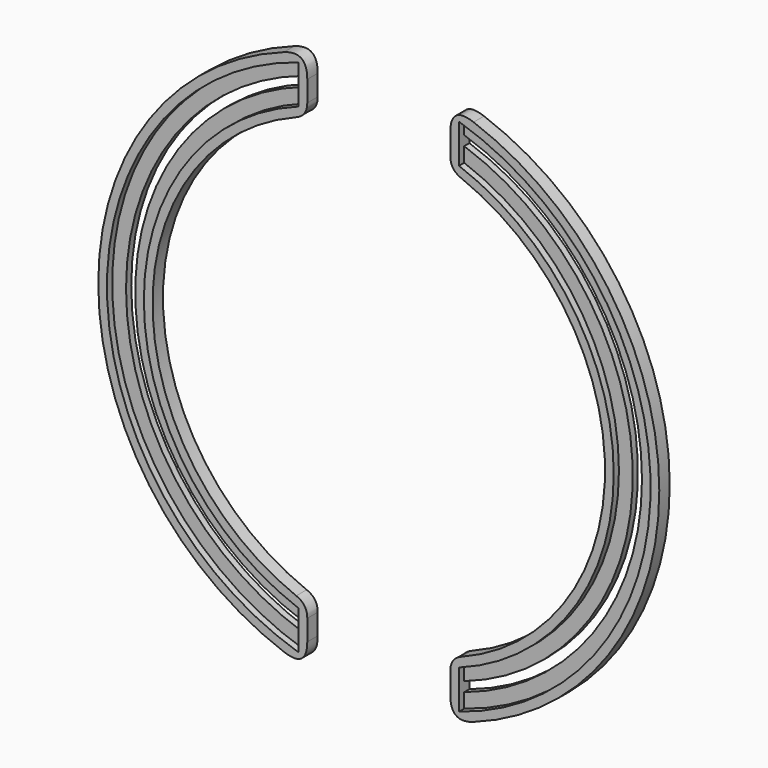
from build123d import *

# Parameters (mm, degrees)
F1_DEPTH      = 1.5
F2_DEPTH      = 3
F3_T1_DEPTH   = 31.0210256648
F3_T3_DEPTH   = 17.0194710076
F3_2_T1_DEPTH = 31.0210256648
F3_2_T3_DEPTH = 17.0194710075


# Not quite as in the source:
# - a fillet or chamfer that OpenCascade refuses, or shapes differently, is made with other operations: its cross-section is extruded or revolved along the edge and cut away or added


with BuildPart() as f1:
    # F0 (on Front) → F1 (new body)
    with BuildSketch(Plane.XZ):
        with BuildLine():
            ThreePointArc((-18.4309218526, 56.3415860789), (-17.4336374643, 56.6581105137), (-16.4309218526, 56.95698385))
            Line((-16.4309218526, 56.95698385), (-16.4309218526, 60.2544953802))
            ThreePointArc((-16.4309218526, 60.2544953802), (-17.433345569, 59.972142439), (-18.4309218526, 59.6731139301))
            Line((-18.4309218526, 59.6731139301), (-18.4309218526, 56.3415860789))
        make_face()
        with BuildLine():
            ThreePointArc((-18.4309218526, -56.3415860789), (-59.2796187759, 0), (-18.4309218526, 56.3415860789))
            Line((-18.4309218526, 56.3415860789), (-18.4309218526, 59.6731139301))
            ThreePointArc((-18.4309218526, 59.6731139301), (-62.4546187759, 0), (-18.4309218526, -59.6731139301))
            Line((-18.4309218526, -59.6731139301), (-18.4309218526, -56.3415860789))
        make_face()
        with BuildLine():
            ThreePointArc((-16.4309218526, -56.95698385), (-17.4336374643, -56.6581105137), (-18.4309218526, -56.3415860789))
            Line((-18.4309218526, -56.3415860789), (-18.4309218526, -59.6731139301))
            ThreePointArc((-18.4309218526, -59.6731139301), (-17.433345569, -59.972142439), (-16.4309218526, -60.2544953802))
            Line((-16.4309218526, -60.2544953802), (-16.4309218526, -56.95698385))
        make_face()
    extrude(amount=F1_DEPTH)



with BuildPart() as f1b:
    # F0 (on Front) → F1, piece 2 (new body)
    with BuildSketch(Plane.XZ):
        with BuildLine():
            ThreePointArc((-18.4309218526, 50.7441040985), (-17.4342611615, 51.0951026895), (-16.4309218526, 51.4265280587))
            Line((-16.4309218526, 51.4265280587), (-16.4309218526, 54.7502492451))
            ThreePointArc((-16.4309218526, 54.7502492451), (-17.4338634076, 54.4391898544), (-18.4309218526, 54.1097597942))
            Line((-18.4309218526, 54.1097597942), (-18.4309218526, 50.7441040985))
        make_face()
        with BuildLine():
            ThreePointArc((-18.4309218526, -50.7441040985), (-53.9876187759, 0), (-18.4309218526, 50.7441040985))
            Line((-18.4309218526, 50.7441040985), (-18.4309218526, 54.1097597942))
            ThreePointArc((-18.4309218526, 54.1097597942), (-57.1626187759, 0), (-18.4309218526, -54.1097597942))
            Line((-18.4309218526, -54.1097597942), (-18.4309218526, -50.7441040985))
        make_face()
        with BuildLine():
            ThreePointArc((-16.4309218526, -51.4265280587), (-17.4342611615, -51.0951026895), (-18.4309218526, -50.7441040985))
            Line((-18.4309218526, -50.7441040985), (-18.4309218526, -54.1097597942))
            ThreePointArc((-18.4309218526, -54.1097597942), (-17.4338634076, -54.4391898544), (-16.4309218526, -54.7502492451))
            Line((-16.4309218526, -54.7502492451), (-16.4309218526, -51.4265280587))
        make_face()
    extrude(amount=F1_DEPTH)


with BuildPart() as f1c:
    # F0 (on Front) → F1, piece 3 (new body)
    with BuildSketch(Plane.XZ):
        with BuildLine():
            ThreePointArc((18.4309218526, -56.3415860789), (17.4336374643, -56.6581105137), (16.4309218526, -56.95698385))
            Line((16.4309218526, -56.95698385), (16.4309218526, -60.2544953802))
            ThreePointArc((16.4309218526, -60.2544953802), (17.433345569, -59.972142439), (18.4309218526, -59.6731139301))
            Line((18.4309218526, -59.6731139301), (18.4309218526, -56.3415860789))
        make_face()
        with BuildLine():
            ThreePointArc((18.4309218526, 56.3415860789), (59.2796187759, 0), (18.4309218526, -56.3415860789))
            Line((18.4309218526, -56.3415860789), (18.4309218526, -59.6731139301))
            ThreePointArc((18.4309218526, -59.6731139301), (62.4546187759, 0), (18.4309218526, 59.6731139301))
            Line((18.4309218526, 59.6731139301), (18.4309218526, 56.3415860789))
        make_face()
        with BuildLine():
            ThreePointArc((16.4309218526, 56.95698385), (17.4336374643, 56.6581105137), (18.4309218526, 56.3415860789))
            Line((18.4309218526, 56.3415860789), (18.4309218526, 59.6731139301))
            ThreePointArc((18.4309218526, 59.6731139301), (17.433345569, 59.972142439), (16.4309218526, 60.2544953802))
            Line((16.4309218526, 60.2544953802), (16.4309218526, 56.95698385))
        make_face()
    extrude(amount=F1_DEPTH)



with BuildPart() as f1d:
    # F0 (on Front) → F1, piece 4 (new body)
    with BuildSketch(Plane.XZ):
        with BuildLine():
            ThreePointArc((18.4309218526, -50.7441040985), (17.4342611615, -51.0951026895), (16.4309218526, -51.4265280587))
            Line((16.4309218526, -51.4265280587), (16.4309218526, -54.7502492451))
            ThreePointArc((16.4309218526, -54.7502492451), (17.4338634076, -54.4391898544), (18.4309218526, -54.1097597942))
            Line((18.4309218526, -54.1097597942), (18.4309218526, -50.7441040985))
        make_face()
        with BuildLine():
            ThreePointArc((18.4309218526, 50.7441040985), (53.9876187759, 0), (18.4309218526, -50.7441040985))
            Line((18.4309218526, -50.7441040985), (18.4309218526, -54.1097597942))
            ThreePointArc((18.4309218526, -54.1097597942), (57.1626187759, 0), (18.4309218526, 54.1097597942))
            Line((18.4309218526, 54.1097597942), (18.4309218526, 50.7441040985))
        make_face()
        with BuildLine():
            ThreePointArc((16.4309218526, 51.4265280587), (17.4342611615, 51.0951026895), (18.4309218526, 50.7441040985))
            Line((18.4309218526, 50.7441040985), (18.4309218526, 54.1097597942))
            ThreePointArc((18.4309218526, 54.1097597942), (17.4338634076, 54.4391898544), (16.4309218526, 54.7502492451))
            Line((16.4309218526, 54.7502492451), (16.4309218526, 51.4265280587))
        make_face()
    extrude(amount=F1_DEPTH)


with BuildPart() as f1_1:
    add(f1.part)

    add(f1b.part)  # F2 merges F1b
    # F0 (on Front) → F2 (join)
    with BuildSketch(Plane.XZ):
        with BuildLine():
            ThreePointArc((-18.4309218526, 59.6731139301), (-17.433345569, 59.972142439), (-16.4309218526, 60.2544953802))
            Line((-16.4309218526, 60.2544953802), (-16.4309218526, 62.3251368921))
            ThreePointArc((-16.4309218526, 62.3251368921), (-17.4331857663, 62.0522514949), (-18.4309218526, 61.7632496005))
            Line((-18.4309218526, 61.7632496005), (-18.4309218526, 59.6731139301))
        make_face()
        with BuildLine():
            ThreePointArc((-18.4309218526, -59.6731139301), (-62.4546187759, 0), (-18.4309218526, 59.6731139301))
            Line((-18.4309218526, 59.6731139301), (-18.4309218526, 61.7632496005))
            ThreePointArc((-18.4309218526, 61.7632496005), (-64.4546187759, 0), (-18.4309218526, -61.7632496005))
            Line((-18.4309218526, -61.7632496005), (-18.4309218526, -59.6731139301))
        make_face()
        with BuildLine():
            ThreePointArc((-16.4309218526, -60.2544953802), (-17.433345569, -59.972142439), (-18.4309218526, -59.6731139301))
            Line((-18.4309218526, -59.6731139301), (-18.4309218526, -61.7632496005))
            ThreePointArc((-18.4309218526, -61.7632496005), (-17.4331857663, -62.0522514949), (-16.4309218526, -62.3251368921))
            Line((-16.4309218526, -62.3251368921), (-16.4309218526, -60.2544953802))
        make_face()
        with BuildLine():
            Line((-16.4309218526, 49.3227869556), (-16.4309218526, 51.4265280587))
            ThreePointArc((-16.4309218526, 51.4265280587), (-17.4342611615, 51.0951026895), (-18.4309218526, 50.7441040985))
            Line((-18.4309218526, 50.7441040985), (-18.4309218526, 48.6108385615))
            ThreePointArc((-18.4309218526, 48.6108385615), (-17.4345563253, 48.9770226916), (-16.4309218526, 49.3227869556))
        make_face()
        with BuildLine():
            Line((-18.4309218526, 48.6108385615), (-18.4309218526, 50.7441040985))
            ThreePointArc((-18.4309218526, 50.7441040985), (-53.9876187759, 0), (-18.4309218526, -50.7441040985))
            Line((-18.4309218526, -50.7441040985), (-18.4309218526, -48.6108385615))
            ThreePointArc((-18.4309218526, -48.6108385615), (-51.9876187759, 0), (-18.4309218526, 48.6108385615))
        make_face()
        with BuildLine():
            Line((-18.4309218526, -48.6108385615), (-18.4309218526, -50.7441040985))
            ThreePointArc((-18.4309218526, -50.7441040985), (-17.4342611615, -51.0951026895), (-16.4309218526, -51.4265280587))
            Line((-16.4309218526, -51.4265280587), (-16.4309218526, -49.3227869556))
            ThreePointArc((-16.4309218526, -49.3227869556), (-17.4345563253, -48.9770226916), (-18.4309218526, -48.6108385615))
        make_face()
        with BuildLine():
            ThreePointArc((-18.4309218526, 54.1097597942), (-17.4338634076, 54.4391898544), (-16.4309218526, 54.7502492451))
            Line((-16.4309218526, 54.7502492451), (-16.4309218526, 56.95698385))
            ThreePointArc((-16.4309218526, 56.95698385), (-17.4336374643, 56.6581105137), (-18.4309218526, 56.3415860789))
            Line((-18.4309218526, 56.3415860789), (-18.4309218526, 54.1097597942))
        make_face()
        with BuildLine():
            ThreePointArc((-18.4309218526, 50.7441040985), (-17.4342611615, 51.0951026895), (-16.4309218526, 51.4265280587))
            Line((-16.4309218526, 51.4265280587), (-16.4309218526, 54.7502492451))
            ThreePointArc((-16.4309218526, 54.7502492451), (-17.4338634076, 54.4391898544), (-18.4309218526, 54.1097597942))
            Line((-18.4309218526, 54.1097597942), (-18.4309218526, 50.7441040985))
        make_face()
        with BuildLine():
            ThreePointArc((-18.4309218526, 56.3415860789), (-17.4336374643, 56.6581105137), (-16.4309218526, 56.95698385))
            Line((-16.4309218526, 56.95698385), (-16.4309218526, 60.2544953802))
            ThreePointArc((-16.4309218526, 60.2544953802), (-17.433345569, 59.972142439), (-18.4309218526, 59.6731139301))
            Line((-18.4309218526, 59.6731139301), (-18.4309218526, 56.3415860789))
        make_face()
        with BuildLine():
            ThreePointArc((-16.4309218526, -51.4265280587), (-17.4342611615, -51.0951026895), (-18.4309218526, -50.7441040985))
            Line((-18.4309218526, -50.7441040985), (-18.4309218526, -54.1097597942))
            ThreePointArc((-18.4309218526, -54.1097597942), (-17.4338634076, -54.4391898544), (-16.4309218526, -54.7502492451))
            Line((-16.4309218526, -54.7502492451), (-16.4309218526, -51.4265280587))
        make_face()
        with BuildLine():
            ThreePointArc((-16.4309218526, -54.7502492451), (-17.4338634076, -54.4391898544), (-18.4309218526, -54.1097597942))
            Line((-18.4309218526, -54.1097597942), (-18.4309218526, -56.3415860789))
            ThreePointArc((-18.4309218526, -56.3415860789), (-17.4336374643, -56.6581105137), (-16.4309218526, -56.95698385))
            Line((-16.4309218526, -56.95698385), (-16.4309218526, -54.7502492451))
        make_face()
        with BuildLine():
            ThreePointArc((-16.4309218526, -56.95698385), (-17.4336374643, -56.6581105137), (-18.4309218526, -56.3415860789))
            Line((-18.4309218526, -56.3415860789), (-18.4309218526, -59.6731139301))
            ThreePointArc((-18.4309218526, -59.6731139301), (-17.433345569, -59.972142439), (-16.4309218526, -60.2544953802))
            Line((-16.4309218526, -60.2544953802), (-16.4309218526, -56.95698385))
        make_face()
    extrude(amount=F2_DEPTH)

    # F3#2: fillet of radius 4 on 4 edges, made by hand

    # F3_2_s2 → F3_2_t1 (cut)
    with BuildSketch(Plane.XZ.offset(-14.0105128324)):
        with BuildLine():
            add(Edge.make_bspline(
                [(-21.7827406063, -60.6622625133), (-16.4309218526, -62.5840055353), (-16.4309218526, -56.8976129869)],
                knots=[0, 0, 0, 1, 1, 1], degree=2, weights=[1, 1, 1]))
            Line((-16.4309218526, -56.8976129869), (-16.4309218526, -62.3251368921))
            ThreePointArc((-16.4309218526, -62.3251368921), (-19.1249127431, -61.5518935056), (-21.7827406063, -60.6622625133))
        make_face()
        with BuildLine():
            add(Edge.make_bspline(
                [(-16.4309218526, 56.8976129868), (-16.4309218526, 62.5840055353), (-21.7827406063, 60.6622625133)],
                knots=[0, 0, 0, 1, 1, 1], degree=2, weights=[1, 1, 1]))
            ThreePointArc((-21.7827406063, 60.6622625133), (-19.1249127431, 61.5518935056), (-16.4309218526, 62.3251368921))
            Line((-16.4309218526, 62.3251368921), (-16.4309218526, 56.8976129868))
        make_face()
    extrude(amount=F3_2_T1_DEPTH, mode=Mode.SUBTRACT)

    # F3_2_s4 → F3_2_t3 (cut)
    with BuildSketch(Plane.XZ.offset(-7.0097355038)):
        with BuildLine():
            add(Edge.make_bspline(
                [(-16.4309218526, -52.1266811571), (-16.4309218526, -49.3981976907), (-18.9712475675, -48.4025234024)],
                knots=[0, 0, 0, 1, 1, 1], degree=2, weights=[1, 1, 1]))
            ThreePointArc((-18.9712475675, -48.4025234024), (-17.7070641599, -48.8791610487), (-16.4309218526, -49.3227869556))
            Line((-16.4309218526, -49.3227869556), (-16.4309218526, -52.1266811571))
        make_face()
        with BuildLine():
            add(Edge.make_bspline(
                [(-16.4309218526, 52.1266811571), (-16.4309218526, 49.3981976907), (-18.9712475675, 48.4025234025)],
                knots=[0, 0, 0, 1, 1, 1], degree=2, weights=[1, 1, 1]))
            ThreePointArc((-18.9712475675, 48.4025234025), (-17.7070641599, 48.8791610487), (-16.4309218526, 49.3227869556))
            Line((-16.4309218526, 49.3227869556), (-16.4309218526, 52.1266811571))
        make_face()
    extrude(amount=F3_2_T3_DEPTH, mode=Mode.SUBTRACT)


with BuildPart() as f1c_1:
    add(f1c.part)

    add(f1d.part)  # F2#2 merges F1d
    # F0 (on Front) → F2, piece 2 (join)
    with BuildSketch(Plane.XZ):
        with BuildLine():
            Line((16.4309218526, -49.3227869556), (16.4309218526, -51.4265280587))
            ThreePointArc((16.4309218526, -51.4265280587), (17.4342611615, -51.0951026895), (18.4309218526, -50.7441040985))
            Line((18.4309218526, -50.7441040985), (18.4309218526, -48.6108385615))
            ThreePointArc((18.4309218526, -48.6108385615), (17.4345563253, -48.9770226916), (16.4309218526, -49.3227869556))
        make_face()
        with BuildLine():
            Line((18.4309218526, -48.6108385615), (18.4309218526, -50.7441040985))
            ThreePointArc((18.4309218526, -50.7441040985), (53.9876187759, 0), (18.4309218526, 50.7441040985))
            Line((18.4309218526, 50.7441040985), (18.4309218526, 48.6108385615))
            ThreePointArc((18.4309218526, 48.6108385615), (51.9876187759, 0), (18.4309218526, -48.6108385615))
        make_face()
        with BuildLine():
            Line((18.4309218526, 48.6108385615), (18.4309218526, 50.7441040985))
            ThreePointArc((18.4309218526, 50.7441040985), (17.4342611615, 51.0951026895), (16.4309218526, 51.4265280587))
            Line((16.4309218526, 51.4265280587), (16.4309218526, 49.3227869556))
            ThreePointArc((16.4309218526, 49.3227869556), (17.4345563253, 48.9770226916), (18.4309218526, 48.6108385615))
        make_face()
        with BuildLine():
            ThreePointArc((18.4309218526, -59.6731139301), (17.433345569, -59.972142439), (16.4309218526, -60.2544953802))
            Line((16.4309218526, -60.2544953802), (16.4309218526, -62.3251368921))
            ThreePointArc((16.4309218526, -62.3251368921), (17.4331857663, -62.0522514949), (18.4309218526, -61.7632496005))
            Line((18.4309218526, -61.7632496005), (18.4309218526, -59.6731139301))
        make_face()
        with BuildLine():
            ThreePointArc((18.4309218526, 59.6731139301), (62.4546187759, 0), (18.4309218526, -59.6731139301))
            Line((18.4309218526, -59.6731139301), (18.4309218526, -61.7632496005))
            ThreePointArc((18.4309218526, -61.7632496005), (64.4546187759, 0), (18.4309218526, 61.7632496005))
            Line((18.4309218526, 61.7632496005), (18.4309218526, 59.6731139301))
        make_face()
        with BuildLine():
            ThreePointArc((16.4309218526, 60.2544953802), (17.433345569, 59.972142439), (18.4309218526, 59.6731139301))
            Line((18.4309218526, 59.6731139301), (18.4309218526, 61.7632496005))
            ThreePointArc((18.4309218526, 61.7632496005), (17.4331857663, 62.0522514949), (16.4309218526, 62.3251368921))
            Line((16.4309218526, 62.3251368921), (16.4309218526, 60.2544953802))
        make_face()
        with BuildLine():
            ThreePointArc((16.4309218526, 54.7502492451), (17.4338634076, 54.4391898544), (18.4309218526, 54.1097597942))
            Line((18.4309218526, 54.1097597942), (18.4309218526, 56.3415860789))
            ThreePointArc((18.4309218526, 56.3415860789), (17.4336374643, 56.6581105137), (16.4309218526, 56.95698385))
            Line((16.4309218526, 56.95698385), (16.4309218526, 54.7502492451))
        make_face()
        with BuildLine():
            ThreePointArc((16.4309218526, 56.95698385), (17.4336374643, 56.6581105137), (18.4309218526, 56.3415860789))
            Line((18.4309218526, 56.3415860789), (18.4309218526, 59.6731139301))
            ThreePointArc((18.4309218526, 59.6731139301), (17.433345569, 59.972142439), (16.4309218526, 60.2544953802))
            Line((16.4309218526, 60.2544953802), (16.4309218526, 56.95698385))
        make_face()
        with BuildLine():
            ThreePointArc((16.4309218526, 51.4265280587), (17.4342611615, 51.0951026895), (18.4309218526, 50.7441040985))
            Line((18.4309218526, 50.7441040985), (18.4309218526, 54.1097597942))
            ThreePointArc((18.4309218526, 54.1097597942), (17.4338634076, 54.4391898544), (16.4309218526, 54.7502492451))
            Line((16.4309218526, 54.7502492451), (16.4309218526, 51.4265280587))
        make_face()
        with BuildLine():
            ThreePointArc((18.4309218526, -54.1097597942), (17.4338634076, -54.4391898544), (16.4309218526, -54.7502492451))
            Line((16.4309218526, -54.7502492451), (16.4309218526, -56.95698385))
            ThreePointArc((16.4309218526, -56.95698385), (17.4336374643, -56.6581105137), (18.4309218526, -56.3415860789))
            Line((18.4309218526, -56.3415860789), (18.4309218526, -54.1097597942))
        make_face()
        with BuildLine():
            ThreePointArc((18.4309218526, -50.7441040985), (17.4342611615, -51.0951026895), (16.4309218526, -51.4265280587))
            Line((16.4309218526, -51.4265280587), (16.4309218526, -54.7502492451))
            ThreePointArc((16.4309218526, -54.7502492451), (17.4338634076, -54.4391898544), (18.4309218526, -54.1097597942))
            Line((18.4309218526, -54.1097597942), (18.4309218526, -50.7441040985))
        make_face()
        with BuildLine():
            ThreePointArc((18.4309218526, -56.3415860789), (17.4336374643, -56.6581105137), (16.4309218526, -56.95698385))
            Line((16.4309218526, -56.95698385), (16.4309218526, -60.2544953802))
            ThreePointArc((16.4309218526, -60.2544953802), (17.433345569, -59.972142439), (18.4309218526, -59.6731139301))
            Line((18.4309218526, -59.6731139301), (18.4309218526, -56.3415860789))
        make_face()
    extrude(amount=F2_DEPTH)

    # F3: fillet of radius 4 on 4 edges, made by hand

    # F3_s2 → F3_t1 (cut)
    with BuildSketch(Plane.XZ.offset(-14.0105128324)):
        with BuildLine():
            add(Edge.make_bspline(
                [(21.7827406063, 60.6622625134), (16.4309218526, 62.5840055354), (16.4309218526, 56.8976129869)],
                knots=[0, 0, 0, 1, 1, 1], degree=2, weights=[1, 1, 1]))
            Line((16.4309218526, 56.8976129869), (16.4309218526, 62.3251368921))
            ThreePointArc((16.4309218526, 62.3251368921), (19.1249127431, 61.5518935056), (21.7827406063, 60.6622625134))
        make_face()
        with BuildLine():
            add(Edge.make_bspline(
                [(16.4309218526, -56.8976129868), (16.4309218526, -62.5840055353), (21.7827406063, -60.6622625133)],
                knots=[0, 0, 0, 1, 1, 1], degree=2, weights=[1, 1, 1]))
            ThreePointArc((21.7827406063, -60.6622625133), (19.1249127431, -61.5518935056), (16.4309218526, -62.3251368921))
            Line((16.4309218526, -62.3251368921), (16.4309218526, -56.8976129868))
        make_face()
    extrude(amount=F3_T1_DEPTH, mode=Mode.SUBTRACT)

    # F3_s4 → F3_t3 (cut)
    with BuildSketch(Plane.XZ.offset(-7.0097355038)):
        with BuildLine():
            add(Edge.make_bspline(
                [(16.4309218526, -52.1266811571), (16.4309218526, -49.3981976907), (18.9712475675, -48.4025234025)],
                knots=[0, 0, 0, 1, 1, 1], degree=2, weights=[1, 1, 1]))
            ThreePointArc((18.9712475675, -48.4025234025), (17.7070641599, -48.8791610487), (16.4309218526, -49.3227869556))
            Line((16.4309218526, -49.3227869556), (16.4309218526, -52.1266811571))
        make_face()
        with BuildLine():
            add(Edge.make_bspline(
                [(16.4309218526, 52.1266811571), (16.4309218526, 49.3981976907), (18.9712475675, 48.4025234024)],
                knots=[0, 0, 0, 1, 1, 1], degree=2, weights=[1, 1, 1]))
            ThreePointArc((18.9712475675, 48.4025234024), (17.7070641599, 48.8791610487), (16.4309218526, 49.3227869556))
            Line((16.4309218526, 49.3227869556), (16.4309218526, 52.1266811571))
        make_face()
    extrude(amount=F3_T3_DEPTH, mode=Mode.SUBTRACT)


solid = Compound([f1_1.part, f1c_1.part])
